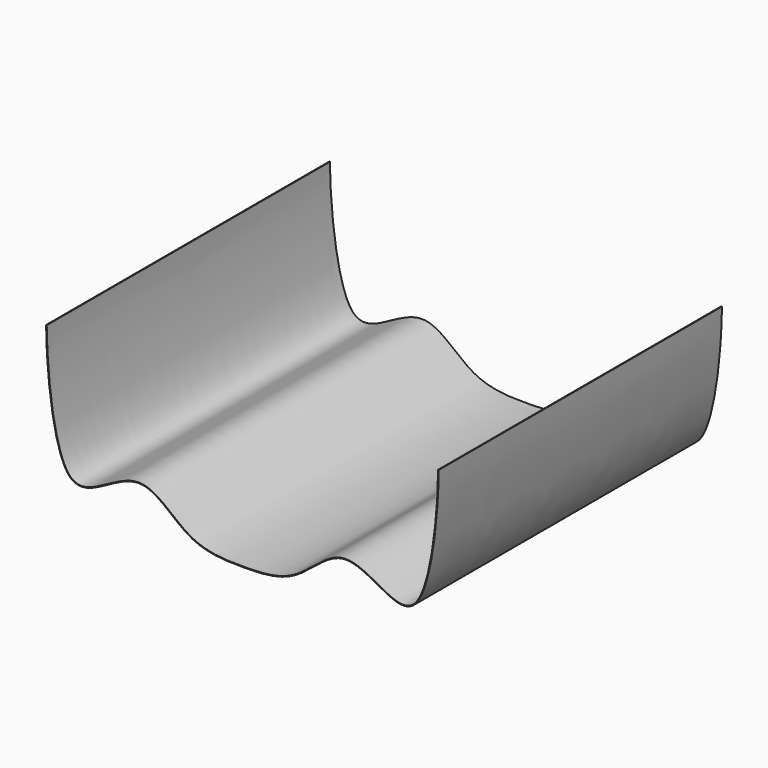
from build123d import *

# Parameters (mm, degrees)
F1_DEPTH = 901.6696214676


# Not quite as in the source:
# - the dataset's text gives a spline's control points without its knots; the knots are read off the source's solid


with BuildPart() as f1:
    # F0 (on Front) → F1 (new body)
    with BuildSketch(Plane.XZ):
        with BuildLine():
            Line((-488.0881249216, 159.1785628277), (-489.6881249216, 159.1785628277))
            add(Edge.make_bspline(
                [(-489.6881249216, 159.1785628277), (-489.6881249216, 75.112275873), (-467.2715724636, -188.5386582623), (-357.9180756465, -171.4212165934), (-240.4726724987, -80.674311093), (-130.040696758, -215.2356028623), (-43.3709902755, -220.8214371723), (10.3118750784, -220.8214371723)],
                knots=[0, 0, 0, 0, 0.2920616724, 0.4305590393, 0.613199573, 0.8067357568, 1, 1, 1, 1], degree=3))
            add(Edge.make_bspline(
                [(510.3118750784, 159.1785628277), (510.3118750784, 75.112275873), (487.8953226204, -188.5386582623), (378.5418258033, -171.4212165934), (261.0964226555, -80.674311093), (150.6644469148, -215.2356028623), (63.9947404323, -220.8214371723), (10.3118750784, -220.8214371723)],
                knots=[0, 0, 0, 0, 0.2920616724, 0.4305590393, 0.613199573, 0.8067357568, 1, 1, 1, 1], degree=3))
            Line((510.3118750784, 159.1785628277), (508.7118750784, 159.1785628277))
            add(Edge.make_bspline(
                [(508.7118750784, 159.1785628277), (508.7118750784, 150.2042864806), (508.3644136442, 130.0777451265), (506.7276009653, 94.9994375448), (503.9031789414, 56.6682889118), (499.8195914315, 16.7180986208), (494.4058845086, -23.2172601205), (487.5924213804, -61.5018157359), (480.6922132126, -90.662947117), (474.4097909677, -111.5203176235), (469.311935055, -125.7189772346), (464.7401446956, -136.1721870406), (460.8907820765, -143.6009921637), (457.9094941962, -148.6785697559), (454.8364761293, -153.2368543326), (451.6758280946, -157.2443619635), (448.4257347578, -160.7158997582), (443.979384374, -164.666664473), (438.2160643259, -168.3972429364), (430.9652792144, -171.1496866876), (423.3498490201, -172.359660341), (412.6887727063, -172.117189677), (401.2885784306, -169.368921953), (389.274936239, -164.7309453896), (376.8965564932, -159.0526054956), (360.8179850439, -150.4478530607), (340.8385374323, -139.2823302839), (323.823866139, -130.5815357657), (310.1044104293, -124.7695055347), (299.7861988422, -121.1833062333), (289.4642609757, -118.5711030047), (280.881057379, -117.3768300602), (274.041244978, -117.1165057188), (268.9300125712, -117.2939590697), (263.8421213882, -117.8759693288), (258.7991534984, -118.859217607), (253.7971445893, -120.2114705565), (247.1803622377, -122.4722811941), (239.0005180001, -126.0889748233), (229.3037651379, -131.4857851383), (216.4960999109, -139.8199964647), (200.6464452143, -151.8726489902), (184.850640247, -164.7862617696), (172.1647094825, -174.8441937117), (162.6076163735, -182.0538064266), (154.5936673057, -187.6189266159), (148.1454670605, -191.7080982615), (143.2882965967, -194.5668578252), (138.400239331, -197.2219107261), (131.8391262275, -200.5016503217), (123.5466395737, -204.1314524951), (113.4235353776, -207.7951933318), (99.6612530327, -211.8358994278), (81.8966053459, -215.449647775), (59.4796584552, -217.9494744103), (35.7723302749, -219.0755731367), (18.9831974416, -219.2214371723), (10.3118750784, -219.2214371723)],
                knots=[0, 0, 0, 0, 0.03125, 0.0625, 0.09375, 0.125, 0.15625, 0.1875, 0.21875, 0.234375, 0.25, 0.265625, 0.2734375, 0.28125, 0.2890625, 0.296875, 0.3046875, 0.3125, 0.328125, 0.34375, 0.359375, 0.375, 0.40625, 0.421875, 0.4375, 0.46875, 0.5, 0.53125, 0.546875, 0.5625, 0.578125, 0.59375, 0.6015625, 0.609375, 0.6171875, 0.625, 0.6328125, 0.640625, 0.65625, 0.671875, 0.6875, 0.71875, 0.75, 0.765625, 0.78125, 0.796875, 0.8046875, 0.8125, 0.8203125, 0.828125, 0.84375, 0.859375, 0.875, 0.90625, 0.9375, 0.96875, 1, 1, 1, 1], degree=3))
            add(Edge.make_bspline(
                [(-488.0881249216, 159.1785628277), (-488.0881249216, 150.2042864806), (-487.7406634874, 130.0777451265), (-486.1038508085, 94.9994375448), (-483.2794287845, 56.6682889118), (-479.1958412746, 16.7180986208), (-473.7821343518, -23.2172601205), (-466.9686712236, -61.5018157359), (-460.0684630557, -90.662947117), (-453.7860408109, -111.5203176235), (-448.6881848982, -125.7189772346), (-444.1163945387, -136.1721870406), (-440.2670319197, -143.6009921637), (-437.2857440393, -148.6785697559), (-434.2127259725, -153.2368543326), (-431.0520779378, -157.2443619635), (-427.801984601, -160.7158997582), (-423.3556342172, -164.666664473), (-417.5923141691, -168.3972429364), (-410.3415290576, -171.1496866876), (-402.7260988633, -172.359660341), (-392.0650225495, -172.117189677), (-380.6648282738, -169.368921953), (-368.6511860822, -164.7309453896), (-356.2728063364, -159.0526054956), (-340.194234887, -150.4478530607), (-320.2147872755, -139.2823302839), (-303.2001159822, -130.5815357657), (-289.4806602725, -124.7695055347), (-279.1624486853, -121.1833062333), (-268.8405108188, -118.5711030047), (-260.2573072222, -117.3768300602), (-253.4174948212, -117.1165057188), (-248.3062624144, -117.2939590697), (-243.2183712313, -117.8759693288), (-238.1754033416, -118.859217607), (-233.1733944325, -120.2114705565), (-226.5566120809, -122.4722811941), (-218.3767678433, -126.0889748233), (-208.6800149811, -131.4857851383), (-195.8723497541, -139.8199964647), (-180.0226950575, -151.8726489902), (-164.2268900901, -164.7862617696), (-151.5409593257, -174.8441937117), (-141.9838662166, -182.0538064266), (-133.9699171488, -187.6189266159), (-127.5217169037, -191.7080982615), (-122.6645464399, -194.5668578252), (-117.7764891742, -197.2219107261), (-111.2153760707, -200.5016503217), (-102.9228894169, -204.1314524951), (-92.7997852208, -207.7951933318), (-79.0375028759, -211.8358994278), (-61.2728551891, -215.449647775), (-38.8559082984, -217.9494744103), (-15.148580118, -219.0755731367), (1.6405527152, -219.2214371723), (10.3118750784, -219.2214371723)],
                knots=[0, 0, 0, 0, 0.03125, 0.0625, 0.09375, 0.125, 0.15625, 0.1875, 0.21875, 0.234375, 0.25, 0.265625, 0.2734375, 0.28125, 0.2890625, 0.296875, 0.3046875, 0.3125, 0.328125, 0.34375, 0.359375, 0.375, 0.40625, 0.421875, 0.4375, 0.46875, 0.5, 0.53125, 0.546875, 0.5625, 0.578125, 0.59375, 0.6015625, 0.609375, 0.6171875, 0.625, 0.6328125, 0.640625, 0.65625, 0.671875, 0.6875, 0.71875, 0.75, 0.765625, 0.78125, 0.796875, 0.8046875, 0.8125, 0.8203125, 0.828125, 0.84375, 0.859375, 0.875, 0.90625, 0.9375, 0.96875, 1, 1, 1, 1], degree=3))
        make_face()
    extrude(amount=F1_DEPTH)


solid = f1.part
